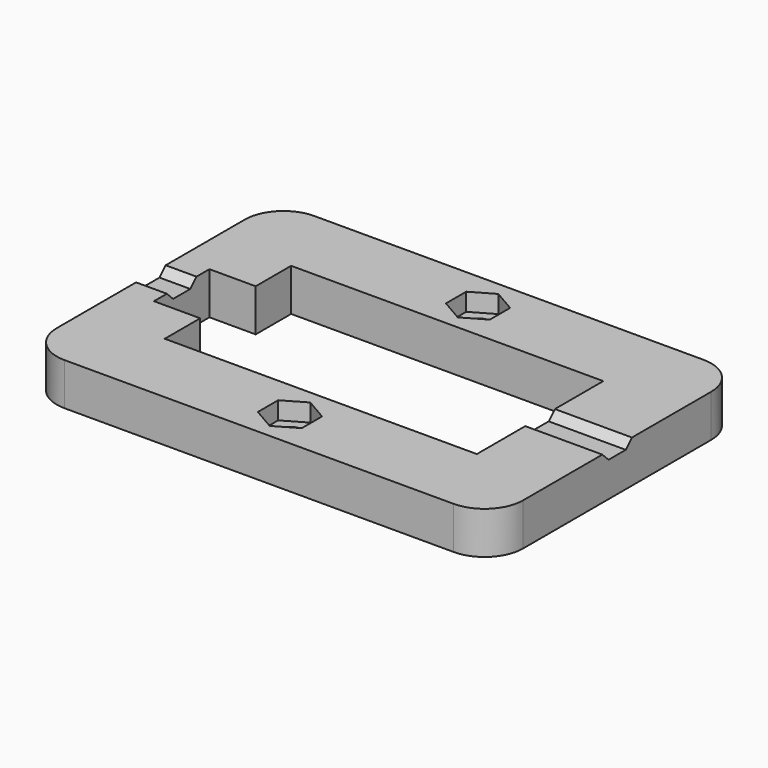
from build123d import *

# Parameters (mm, degrees)
F0_W     = 60.5
F0_H     = 40.5
F0_W_2   = 40.5
F0_H_2   = 20.5
F1_DEPTH = 5.5
F2_W     = 10
F2_H     = 2.8
F3_DEPTH = 1
F4_R     = 1.65
F5_DEPTH = 25
F6_W     = 6
F6_H     = 9
F7_DEPTH = 25
F9_DEPTH = 2.3
F10_SIZE = 0.99999
F11_R    = 5


# Not quite as in the source:
# - a fillet or chamfer is up to 0.001 mm smaller than in the source, because OpenCascade refuses the exact size


with BuildPart() as f1:
    # F0 (on Top) → F1 (new body)
    with BuildSketch(Plane.XY):
        Rectangle(F0_W, F0_H)
        Rectangle(F0_W_2, F0_H_2, mode=Mode.SUBTRACT)
    extrude(amount=F1_DEPTH)

    # F2 (on face) → F3 (cut)
    with BuildSketch(Plane.XY.offset(5.5)):
        with Locations((-25.25, 0)):
            Rectangle(F2_W, F2_H)
        with Locations((25.25, 0)):
            Rectangle(F2_W, F2_H)
    extrude(amount=-F3_DEPTH, mode=Mode.SUBTRACT)

    # F4 (on face) → F5 (cut)
    with BuildSketch(Plane.XY.offset(5.5)):
        with Locations((0, 15.25)):
            Circle(F4_R)
        with Locations((0, -15.25)):
            Circle(F4_R)
    extrude(amount=-F5_DEPTH, mode=Mode.SUBTRACT)

    # F6 (on face) → F7 (cut)
    with BuildSketch(Plane(origin=(0, 0, 0), x_dir=(1, 0, 0), z_dir=(0, 0, -1))):
        with Locations((-23.25, 0)):
            Rectangle(F6_W, F6_H)
    extrude(amount=-F7_DEPTH, mode=Mode.SUBTRACT)

    # F8 (on face) → F9 (cut)
    with BuildSketch(Plane.XY.offset(5.5)):
        Polygon((2.85, 13.6045517328), (2.85, 16.8954482672), (0, 18.5408965344), (-2.85, 16.8954482672), (-2.85, 13.6045517328), (0, 11.9591034656), align=None)
        Polygon((-2.85, -16.8954482672), (0, -18.5408965344), (2.85, -16.8954482672), (2.85, -13.6045517328), (0, -11.9591034656), (-2.85, -13.6045517328), align=None)
    extrude(amount=-F9_DEPTH, mode=Mode.SUBTRACT)

    # F10 (size 1 in the source; OpenCascade refuses exactly that, so slightly less here)
    f10_edges = [f1.edges().sort_by_distance(p)[0] for p in [
        (25.25, 1.4, 5.5),
        (25.25, -1.4, 5.5),
        (-28.25, 1.4, 5.5),
        (-28.25, -1.4, 5.5),
    ]]
    chamfer(f10_edges, length=F10_SIZE)

    # F11
    f11_edges = [f1.edges().sort_by_distance(p)[0] for p in [
        (30.25, 20.25, 2.75),
        (30.25, -20.25, 2.75),
        (-30.25, -20.25, 2.75),
        (-30.25, 20.25, 2.75),
    ]]
    fillet(f11_edges, radius=F11_R)


solid = f1.part
